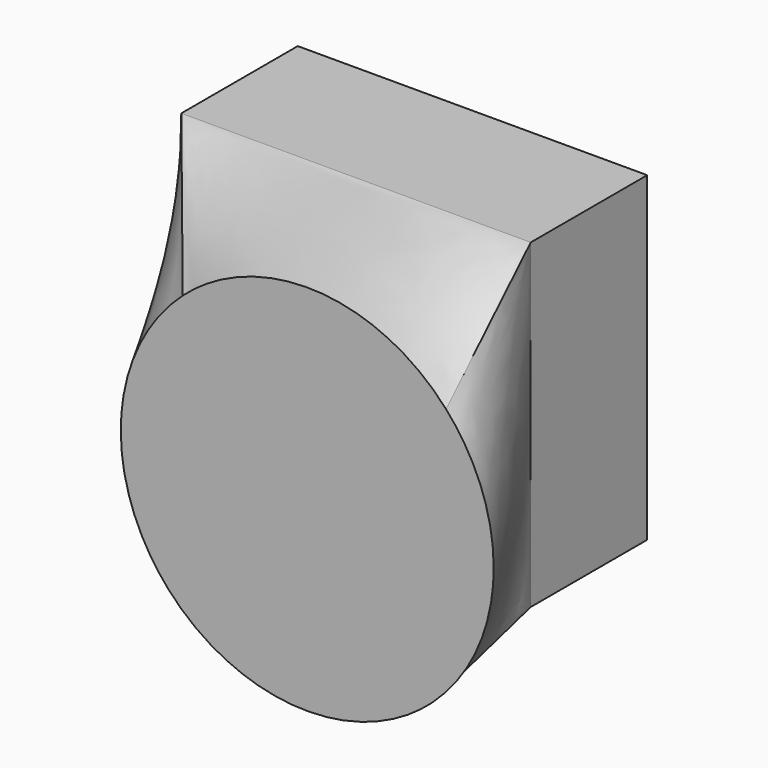
from build123d import *

# Parameters (mm, degrees)
F0_W      = 60
F0_H      = 55.1169423331
F1_DEPTH  = 25
F1_FACE_W = 60
F1_FACE_H = 55.1169423331


# Not quite as in the source:
# - the arcs of a loft's sections are written as splines that run evenly, so that the points pair up as in the source's solid


with BuildPart() as f1:
    # F0 (on Front) → F1 (new body)
    with BuildSketch(Plane.XZ):
        Rectangle(F0_W, F0_H)
    extrude(amount=F1_DEPTH)


with BuildPart() as f4:
    # F1_face (on face) → F4 section 0
    with BuildSketch(Plane.XZ.offset(25)):
        Rectangle(F1_FACE_W, F1_FACE_H)
    # F3 (on offset) → F4 section 1
    with BuildSketch(Plane.XZ.offset(50)):
        with BuildLine():
            add(Edge.make_bspline(
                [(33.0049454892, -30.9087265839), (34.5648464401, -29.509604206), (35.9869107002, -27.9568833895), (38.5008560126, -24.6037629645), (39.5926749027, -22.8034462686), (41.4041541174, -19.0243087118), (42.1237696497, -17.0455812976), (43.1631686363, -12.985656746), (43.4829263895, -10.9045599983), (43.7103016279, -6.7198690755), (43.6179134909, -4.6163783752), (43.0245270782, -0.4677364066), (42.5235434753, 1.5773122783), (41.1321989185, 5.5304753085), (40.2418723685, 7.4384919039), (38.1060382588, 11.0442581573), (36.8605835118, 12.7419186555), (35.4614611339, 14.3018196063)],
                knots=[0, 0, 0, 0, 0.125, 0.125, 0.25, 0.25, 0.375, 0.375, 0.5, 0.5, 0.625, 0.625, 0.75, 0.75, 0.875, 0.875, 1, 1, 1, 1], degree=3))
            add(Edge.make_bspline(
                [(35.4614611339, 14.3018196063), (34.0623387561, 15.8617205572), (32.5096179395, 17.2837848173), (29.1564975146, 19.7977301297), (27.3561808187, 20.8895490198), (23.5770432619, 22.7010282345), (21.5983158477, 23.4206437668), (17.5383912961, 24.4600427534), (15.4572945483, 24.7798005066), (11.2726036256, 25.0071757451), (9.1691129253, 24.914787608), (5.0204709567, 24.3214011953), (2.9754222718, 23.8204175924), (-0.9777407584, 22.4290730356), (-2.8857573538, 21.5387464856), (-6.4915236072, 19.4029123759), (-8.1891841054, 18.1574576289), (-9.7490850563, 16.7583352511)],
                knots=[0, 0, 0, 0, 0.125, 0.125, 0.25, 0.25, 0.375, 0.375, 0.5, 0.5, 0.625, 0.625, 0.75, 0.75, 0.875, 0.875, 1, 1, 1, 1], degree=3))
            add(Edge.make_bspline(
                [(-9.7490850563, 16.7583352511), (-11.3089860071, 15.3592128732), (-12.7310502672, 13.8064920567), (-15.2449955797, 10.4533716317), (-16.3368144697, 8.6530549358), (-18.1482936844, 4.873917379), (-18.8679092167, 2.8951899648), (-19.9073082033, -1.1647345868), (-20.2270659565, -3.2458313345), (-20.454441195, -7.4305222573), (-20.3620530579, -9.5340129576), (-19.7686666453, -13.6826549262), (-19.2676830423, -15.7277036111), (-17.8763384856, -19.6808666413), (-16.9860119356, -21.5888832367), (-14.8501778258, -25.1946494901), (-13.6047230788, -26.8923099883), (-12.205600701, -28.4522109391)],
                knots=[0, 0, 0, 0, 0.125, 0.125, 0.25, 0.25, 0.375, 0.375, 0.5, 0.5, 0.625, 0.625, 0.75, 0.75, 0.875, 0.875, 1, 1, 1, 1], degree=3))
            add(Edge.make_bspline(
                [(-12.205600701, -28.4522109391), (-10.8064783231, -30.01211189), (-9.2537575066, -31.4341761501), (-5.9006370816, -33.9481214625), (-4.1003203857, -35.0399403526), (-0.321182829, -36.8514195673), (1.6575445853, -37.5710350996), (5.7174691369, -38.6104340862), (7.7985658846, -38.9301918394), (11.9832568074, -39.1575670779), (14.0867475077, -39.0651789408), (18.2353894763, -38.4717925281), (20.2804381612, -37.9708089252), (24.2336011913, -36.5794643685), (26.1416177868, -35.6891378184), (29.7473840402, -33.5533037087), (31.4450445384, -32.3078489617), (33.0049454892, -30.9087265839)],
                knots=[0, 0, 0, 0, 0.125, 0.125, 0.25, 0.25, 0.375, 0.375, 0.5, 0.5, 0.625, 0.625, 0.75, 0.75, 0.875, 0.875, 1, 1, 1, 1], degree=3))
        make_face()
    loft(ruled=True)


solid = Compound([f1.part, f4.part])
